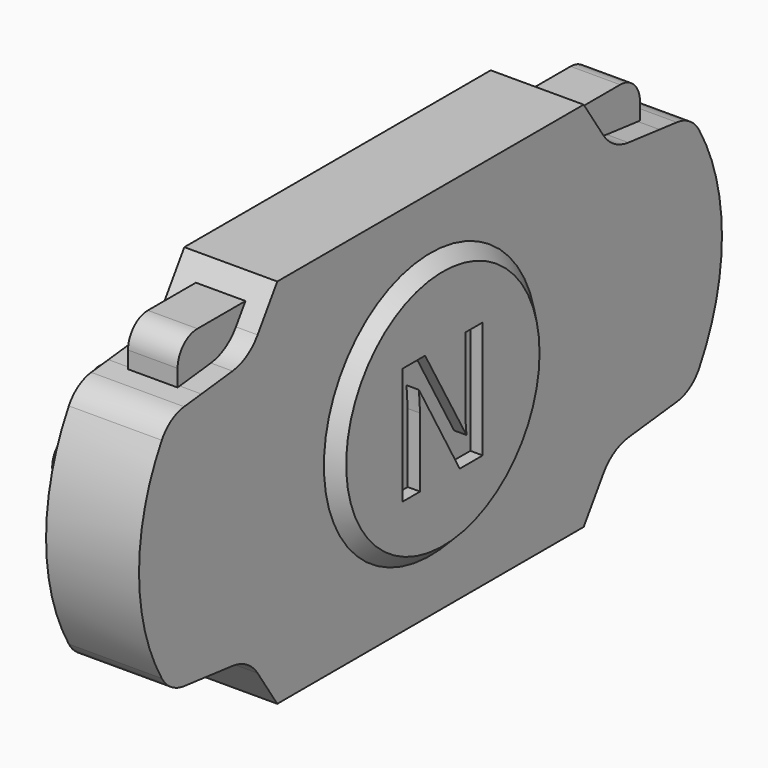
from build123d import *

# Parameters (mm, degrees)
F1_DEPTH      = 7.5
F3_DEPTH      = 4
F4_W          = 60
F4_H          = 35
F5_DEPTH      = 2
F6_R          = 3.5
F7_DEPTH      = 3
F8_R          = 2
F9_R          = 22.5
F10_DEPTH     = 2
F12_TEXT_SIZE = 27.4697590309
F13_DEPTH     = 2
F15_DEPTH     = 2
F15_TAPER     = 5
F16_TEXT_SIZE = 10.8366961487
F17_DEPTH     = 2
F25_R         = 3
F26_DEPTH     = 3
F27_R         = 5
F28_DEPTH     = 3
F30_W         = 3.5
F30_H         = 3.5
F30_W_2       = 3
F30_H_2       = 3
F31_DEPTH     = 2
F32_R         = 1.9688211253
F32_R_2       = 1.5
F33_DEPTH     = 2
F35_DEPTH     = 2
F37_DEPTH     = 2
F39_DEPTH     = 2
F41_R         = 1.75
F42_DEPTH     = 20
F44_DEPTH     = 10


# Not quite as in the source:
# - a fillet or chamfer that OpenCascade refuses, or shapes differently, is made with other operations: its cross-section is extruded or revolved along the edge and cut away or added
# - Text() gives the source's letters only with a copy of the font that has no kerning and outlines rounded to 1/6400 em; it was checked with that copy


with BuildPart() as f1:
    # F0 (on Right) → F1 (new body, symmetric)
    with BuildSketch(Plane.YZ):
        with BuildLine():
            Line((-34.8711436077, -24.0259013658), (-30.9017617255, -30))
            Line((-30.9017617255, -30), (0, -30))
            Line((0, -30), (0, 0))
            Line((0, 0), (-52.5, 0))
            Line((-52.5, 0), (-52.5, -18.7762488504))
            ThreePointArc((-52.5, -18.7762488504), (-51.1634624835, -19.4917800985), (-49.6902439515, -19.8494736223))
            Line((-49.6902439515, -19.8494736223), (-46.2112579103, -20.2390480822))
            Line((-46.2112579103, -20.2390480822), (-39.9225158206, -20.9432570884))
            ThreePointArc((-39.9225158206, -20.9432570884), (-37.0550608987, -21.9245400717), (-34.8711436077, -24.0259013658))
        make_face()
        with BuildLine():
            Line((0, 0), (0, -30))
            Line((0, -30), (30.9017617255, -30))
            Line((30.9017617255, -30), (34.8711436077, -24.0259013658))
            ThreePointArc((34.8711436077, -24.0259013658), (37.0550608987, -21.9245400717), (39.9225158206, -20.9432570884))
            Line((39.9225158206, -20.9432570884), (46.2112579103, -20.2390480822))
            Line((46.2112579103, -20.2390480822), (49.6902439515, -19.8494736223))
            ThreePointArc((49.6902439515, -19.8494736223), (51.1634624835, -19.4917800985), (52.5, -18.7762488504))
            Line((52.5, -18.7762488504), (52.5, 0))
            Line((52.5, 0), (0, 0))
        make_face()
        with BuildLine():
            Line((-52.5, 0), (0, 0))
            Line((0, 0), (0, 30))
            Line((0, 30), (-30.9017617255, 30))
            Line((-30.9017617255, 30), (-34.8711436077, 24.0259013658))
            ThreePointArc((-34.8711436077, 24.0259013658), (-37.0550608987, 21.9245400717), (-39.9225158206, 20.9432570884))
            Line((-39.9225158206, 20.9432570884), (-46.2112579103, 20.2390480822))
            Line((-46.2112579103, 20.2390480822), (-49.6902439515, 19.8494736223))
            ThreePointArc((-49.6902439515, 19.8494736223), (-51.1634624835, 19.4917800985), (-52.5, 18.7762488504))
            Line((-52.5, 18.7762488504), (-52.5, 0))
        make_face()
        with BuildLine():
            Line((0, 30), (0, 0))
            Line((0, 0), (52.5, 0))
            Line((52.5, 0), (52.5, 18.7762488504))
            ThreePointArc((52.5, 18.7762488504), (51.1634624835, 19.4917800985), (49.6902439515, 19.8494736223))
            Line((49.6902439515, 19.8494736223), (46.2112579103, 20.2390480822))
            Line((46.2112579103, 20.2390480822), (39.9225158206, 20.9432570884))
            ThreePointArc((39.9225158206, 20.9432570884), (37.0550608987, 21.9245400717), (34.8711436077, 24.0259013658))
            Line((34.8711436077, 24.0259013658), (30.9017617255, 30))
            Line((30.9017617255, 30), (0, 30))
        make_face()
        with BuildLine():
            Line((58.7885477615, 0), (52.5, 0))
            Line((52.5, 0), (52.5, -18.7762488504))
            ThreePointArc((52.5, -18.7762488504), (53.448824854, -17.9374222983), (54.2004466552, -16.9181268278))
            ThreePointArc((54.2004466552, -16.9181268278), (57.6211742241, -8.7646119013), (58.7885477615, 0))
        make_face()
        with BuildLine():
            Line((52.5, 18.7762488504), (52.5, 0))
            Line((52.5, 0), (58.7885477615, 0))
            ThreePointArc((58.7885477615, 0), (57.6211742241, 8.7646119013), (54.2004466552, 16.9181268278))
            ThreePointArc((54.2004466552, 16.9181268278), (53.448824854, 17.9374222983), (52.5, 18.7762488504))
        make_face()
        with BuildLine():
            Line((-58.7885477615, 0), (-52.5, 0))
            Line((-52.5, 0), (-52.5, 18.7762488504))
            ThreePointArc((-52.5, 18.7762488504), (-53.448824854, 17.9374222983), (-54.2004466552, 16.9181268278))
            ThreePointArc((-54.2004466552, 16.9181268278), (-57.6211742241, 8.7646119013), (-58.7885477615, 0))
        make_face()
        with BuildLine():
            Line((-52.5, -18.7762488504), (-52.5, 0))
            Line((-52.5, 0), (-58.7885477615, 0))
            ThreePointArc((-58.7885477615, 0), (-57.6211742241, -8.7646119013), (-54.2004466552, -16.9181268278))
            ThreePointArc((-54.2004466552, -16.9181268278), (-53.448824854, -17.9374222983), (-52.5, -18.7762488504))
        make_face()
    extrude(amount=F1_DEPTH, both=True)

    # F2 (on Right) → F3 (join, symmetric)
    with BuildSketch(Plane.YZ):
        with BuildLine():
            Line((29.7115407884, 26.9230790436), (29.7115407884, 18.846154213))
            Line((29.7115407884, 18.846154213), (46.6346181929, 18.846154213))
            Line((46.6346181929, 18.846154213), (46.6346181929, 22.9230790436))
            ThreePointArc((46.6346181929, 22.9230790436), (45.4630453177, 25.7515061684), (42.6346181929, 26.9230790436))
            Line((42.6346181929, 26.9230790436), (29.7115407884, 26.9230790436))
        make_face()
        with BuildLine():
            Line((-29.7115407884, 18.846154213), (-29.7115407884, 26.9230790436))
            Line((-29.7115407884, 26.9230790436), (-42.6346181929, 26.9230790436))
            ThreePointArc((-42.6346181929, 26.9230790436), (-45.4630453177, 25.7515061684), (-46.6346181929, 22.9230790436))
            Line((-46.6346181929, 22.9230790436), (-46.6346181929, 18.846154213))
            Line((-46.6346181929, 18.846154213), (-29.7115407884, 18.846154213))
        make_face()
    extrude(amount=F3_DEPTH, both=True)

    # F4 (on face) → F5 (cut)
    with BuildSketch(Plane(origin=(-7.5, 0, 0), x_dir=(0, -1, 0), z_dir=(-1, 0, 0))):
        Rectangle(F4_W, F4_H)
    extrude(amount=-F5_DEPTH, mode=Mode.SUBTRACT)

    # F6 (on face) → F7 (join)
    with BuildSketch(Plane(origin=(-7.5, 0, 0), x_dir=(0, -1, 0), z_dir=(-1, 0, 0))):
        with BuildLine():
            ThreePointArc((-40.8078288883, 14.117408731), (-46.7827026225, 16.5922824652), (-44.3078288883, 10.617408731))
            ThreePointArc((-44.3078288883, 10.617408731), (-41.8329551542, 11.6425349969), (-40.8078288883, 14.117408731))
        make_face()
        with BuildLine():
            ThreePointArc((-34.8078288883, 7.117408731), (-38.3078288883, 10.617408731), (-41.8078288883, 7.117408731))
            ThreePointArc((-41.8078288883, 7.117408731), (-38.3078288883, 3.617408731), (-34.8078288883, 7.117408731))
        make_face()
        with BuildLine():
            ThreePointArc((-40.8078288883, 0.117408731), (-41.8329551542, 2.5922824652), (-44.3078288883, 3.617408731))
            ThreePointArc((-44.3078288883, 3.617408731), (-46.7827026225, -2.3574650031), (-40.8078288883, 0.117408731))
        make_face()
        with Locations((-50.3078288883, 7.117408731)):
            Circle(F6_R)
        with Locations((44.3078288883, 14.117408731)):
            Circle(F6_R)
        with Locations((38.3078288883, 7.117408731)):
            Circle(F6_R)
        with Locations((44.3078288883, 0.117408731)):
            Circle(F6_R)
        with Locations((50.3078288883, 7.117408731)):
            Circle(F6_R)
    extrude(amount=F7_DEPTH)

    # F8
    f8_edges = [f1.edges().sort_by_distance(p)[0] for p in [
        (-10.5, 44.307829, 17.617409),
        (-10.5, 34.807829, 7.117409),
        (-10.5, 44.307829, -3.382591),
        (-10.5, 53.807829, 7.117409),
    ]]
    fillet(f8_edges, radius=F8_R)

    # F9 (on face) → F10 (join)
    with BuildSketch(Plane.YZ.offset(7.5)):
        Circle(F9_R)
    extrude(amount=F10_DEPTH)

    # F11: chamfer of 3 on 1 edges, made by hand


with BuildPart() as f11_tool2:
    # F11_s3 → F11_t4 (revolve)
    with BuildSketch(Plane.XY):
        Polygon((6.5, 22.5), (9.5, 19.5), (9.5, 22.5), align=None)
    revolve(axis=Axis((9.5, 0, 0), (1, 0, 0)))

    split(bisect_by=Plane.YZ.offset(7.5), keep=Keep.TOP)


with BuildPart() as f1_1:
    add(f1.part)

    # F11_t1: cut F11_tool2
    add(f11_tool2.part, mode=Mode.SUBTRACT)

    # F12 (on face) → F13 (cut)
    with BuildSketch(Plane.YZ.offset(9.5)):
        with Locations((-9.9470572741, -9.8891132511)):
            Text('N', F12_TEXT_SIZE, font='Arimo', font_style=FontStyle.BOLD, text_align=(TextAlign.LEFT, TextAlign.BOTTOM))
    extrude(amount=-F13_DEPTH, mode=Mode.SUBTRACT)

    # F14 (on face) → F15 (join)
    with BuildSketch(Plane(origin=(-7.5, 0, 0), x_dir=(0, -1, 0), z_dir=(-1, 0, 0))):
        with BuildLine():
            Line((-29.8438798379, -25.3125000745), (-20.5795092393, -25.3125000745))
            ThreePointArc((-20.5795092393, -25.3125000745), (-19.8724024581, -25.0196068557), (-19.5795092393, -24.3125000745))
            ThreePointArc((-19.5795092393, -24.3125000745), (-19.8724024581, -23.6053932933), (-20.5795092393, -23.3125000745))
            Line((-20.5795092393, -23.3125000745), (-29.8438798379, -23.3125000745))
            ThreePointArc((-29.8438798379, -23.3125000745), (-30.5509866191, -23.6053932933), (-30.8438798379, -24.3125000745))
            ThreePointArc((-30.8438798379, -24.3125000745), (-30.5509866191, -25.0196068557), (-29.8438798379, -25.3125000745))
        make_face()
    extrude(amount=F15_DEPTH, taper=F15_TAPER)

    # F16 (on face) → F17 (cut)
    with BuildSketch(Plane(origin=(-7.5, 0, 0), x_dir=(0, -1, 0), z_dir=(-1, 0, 0))):
        with Locations((-4.2694889592, 19.8689512908)):
            Text('N', F16_TEXT_SIZE, font='Open Sans', font_style=FontStyle.BOLD, text_align=(TextAlign.LEFT, TextAlign.BOTTOM))
    extrude(amount=-F17_DEPTH, mode=Mode.SUBTRACT)

    # F19 (on offset) → F20 (revolve, cut)
    with BuildSketch(Plane.YZ.offset(-4.5)):
        with BuildLine():
            ThreePointArc((43.8205674291, -15.9778223559), (47.356101335, -14.5133562619), (48.8205674291, -10.9778223559))
            ThreePointArc((48.8205674291, -10.9778223559), (47.3576538302, -7.4438416272), (43.8249595128, -5.977824285))
            Line((43.8249595128, -5.977824285), (43.8205674291, -15.9778223559))
        make_face()
    revolve(axis=Axis((-4.5, 43.8227634709, -10.9778233204), (0, -0.0004392084, -0.9999999035)), mode=Mode.SUBTRACT)

    # F30 (on face) → F31 (cut)
    with BuildSketch(Plane(origin=(-10.5, 0, 0), x_dir=(0, -1, 0), z_dir=(-1, 0, 0))):
        with Locations((38.3078288883, 7.117408731)):
            Rectangle(F30_W, F30_H)
        with Locations((38.3078288883, 7.117408731)):
            Rectangle(F30_W_2, F30_H_2, mode=Mode.SUBTRACT)
    extrude(amount=-F31_DEPTH, mode=Mode.SUBTRACT)

    # F32 (on face) → F33 (cut)
    with BuildSketch(Plane(origin=(-10.5, 0, 0), x_dir=(0, -1, 0), z_dir=(-1, 0, 0))):
        with Locations((50.3078288883, 7.117408731)):
            Circle(F32_R)
        with Locations((50.3078288883, 7.117408731)):
            Circle(F32_R_2, mode=Mode.SUBTRACT)
    extrude(amount=-F33_DEPTH, mode=Mode.SUBTRACT)

    # F34 (on face) → F35 (join)
    with BuildSketch(Plane(origin=(-10.5, 0, 0), x_dir=(0, -1, 0), z_dir=(-1, 0, 0))):
        Polygon((42.4578288883, 13.049310733), (46.1578288883, 13.049310733), (44.3078288883, 16.253604727), align=None)
        Polygon((42.8619163417, 13.282610733), (44.3078288883, 15.787004727), (45.7537414349, 13.282610733), align=None, mode=Mode.SUBTRACT)
    extrude(amount=-F35_DEPTH)

    # F36 (on face) → F37 (cut)
    with BuildSketch(Plane(origin=(-10.5, 0, 0), x_dir=(0, -1, 0), z_dir=(-1, 0, 0))):
        Polygon((42.4578288883, 13.049310733), (46.1578288883, 13.049310733), (44.3078288883, 16.253604727), align=None)
        Polygon((44.3078288883, 15.8494595386), (45.8078288883, 13.2513833272), (42.8078288883, 13.2513833272), align=None, mode=Mode.SUBTRACT)
    extrude(amount=-F37_DEPTH, mode=Mode.SUBTRACT)

    # F38 (on face) → F39 (cut)
    with BuildSketch(Plane(origin=(-10.5, 0, 0), x_dir=(0, -1, 0), z_dir=(-1, 0, 0))):
        Polygon((45.3543469245, -1.4523683232), (45.8776059426, -0.9291093051), (44.8310879064, 0.117408731), (45.8776059426, 1.1639267672), (45.3543469245, 1.6871857853), (44.3078288883, 0.6406677491), (43.2613108522, 1.6871857853), (42.7380518341, 1.1639267672), (43.7845698702, 0.117408731), (42.7380518341, -0.9291093051), (43.2613108522, -1.4523683232), (44.3078288883, -0.405850287), align=None)
    extrude(amount=-F39_DEPTH, mode=Mode.SUBTRACT)

    # F41 (on offset) → F42 (cut)
    with BuildSketch(Plane.XZ.offset(-40)):
        with Locations((0, -24.5135370642)):
            Circle(F41_R)
    extrude(amount=F42_DEPTH, mode=Mode.SUBTRACT)

    # F43 (on face) → F44 (cut)
    with BuildSketch(Plane(origin=(0, 0, -30), x_dir=(1, 0, 0), z_dir=(0, 0, -1))):
        with BuildLine():
            ThreePointArc((-1.0266593135, 26.0873075647), (-1.2251112764, 26.1516440057), (-1.4325933487, 26.1734051853))
            Line((-1.4325933487, 26.1734051853), (-1.8108805334, 26.1734051853))
            ThreePointArc((-1.8108805334, 26.1734051853), (-2.5179873146, 25.8805119665), (-2.8108805334, 25.1734051853))
            Line((-2.8108805334, 25.1734051853), (-2.8108805334, 17.1734051853))
            ThreePointArc((-2.8108805334, 17.1734051853), (-2.5179873146, 16.4662984042), (-1.8108805334, 16.1734051853))
            Line((-1.8108805334, 16.1734051853), (-1.4325933487, 16.1734051853))
            ThreePointArc((-1.4325933487, 16.1734051853), (-1.2251112764, 16.195166365), (-1.0266593135, 16.2595028059))
            Line((-1.0266593135, 16.2595028059), (1.5950535018, 17.4240062434))
            ThreePointArc((1.5950535018, 17.4240062434), (2.0275507504, 17.7929012995), (2.1891194666, 18.3379086228))
            Line((2.1891194666, 18.3379086228), (2.1891194666, 24.0089017479))
            ThreePointArc((2.1891194666, 24.0089017479), (2.0275507504, 24.5539090712), (1.5950535018, 24.9228041273))
            Line((1.5950535018, 24.9228041273), (-1.0266593135, 26.0873075647))
        make_face()
    extrude(amount=-F44_DEPTH, mode=Mode.SUBTRACT)


with BuildPart() as f23:
    # F22 (on offset) → F23 (revolve)
    with BuildSketch(Plane.YZ.offset(-4.5)):
        with BuildLine():
            ThreePointArc((43.818987906, -14.9237330034), (46.6474150307, -13.7521601282), (47.818987906, -10.9237330034))
            ThreePointArc((47.818987906, -10.9237330034), (46.6474150307, -8.0953058787), (43.818987906, -6.9237330034))
            Line((43.818987906, -6.9237330034), (43.818987906, -14.9237330034))
        make_face()
    revolve(axis=Axis((-4.5, 43.818987906, -11.1819556914), (0, 0, -1)))

    # F25 (on offset) → F26 (join)
    with BuildSketch(Plane.YZ.offset(-7)):
        with Locations((43.8205674291, -10.9925409779)):
            Circle(F25_R)
    extrude(amount=-F26_DEPTH)

    # F27 (on face) → F28 (join)
    with BuildSketch(Plane(origin=(-10, 0, 0), x_dir=(0, -1, 0), z_dir=(-1, 0, 0))):
        with Locations((-43.8205674291, -10.9925409779)):
            Circle(F27_R)
    extrude(amount=F28_DEPTH)

    # F29: fillet of radius 5 on 1 edges, made by hand

    # F29_s1 → F29_t2 (revolve, cut)
    with BuildSketch(Plane.XY.offset(-10.9925409779)):
        with BuildLine():
            ThreePointArc((-10, 38.8205674291), (-12.1833001327, 40.6645303365), (-13, 43.403143124))
            Line((-13, 43.403143124), (-13, 38.8205674291))
            Line((-13, 38.8205674291), (-10, 38.8205674291))
        make_face()
    revolve(axis=Axis((-13, 43.8205674291, -10.9925409779), (-1, 0, 0)), mode=Mode.SUBTRACT)


solid = Compound([f1_1.part, f23.part])
